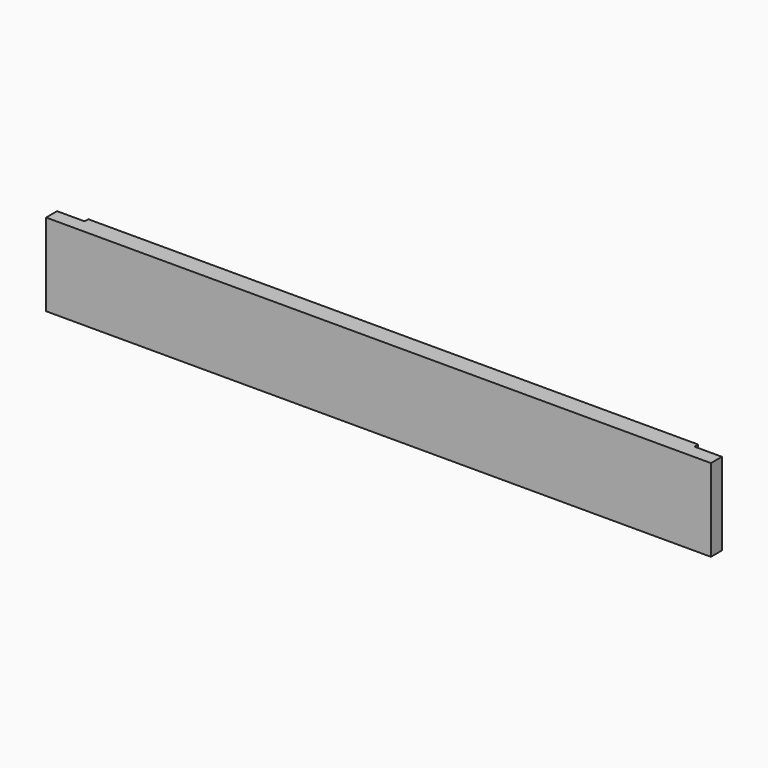
from build123d import *

# Parameters (mm, degrees)
F1_DEPTH      = 230.1875
F2_W          = 19.05
F2_H          = 9.525
F3_DEPTH      = 493
F3_DEPTH_BACK = 57.151


# Not quite as in the source:
# - an extrude ends at something that could not be found from the text; its depth is read off the source's solid


with BuildPart() as f1:
    # F0 (on Right) → F1 (new body, symmetric)
    with BuildSketch(Plane.YZ):
        Polygon((-19.05, 57.15), (-19.05, 0), (0, 0), (0, 38.1), (-6.35, 38.1), (-6.35, 57.15), align=None)
    extrude(amount=F1_DEPTH, both=True)

    # F2 (on Top) → F3 (cut, two sides)
    with BuildSketch(Plane.XY) as f3_sk:
        with Locations((220.6625, -4.7625)):
            Rectangle(F2_W, F2_H)
        with Locations((-220.6625, -4.7625)):
            Rectangle(F2_W, F2_H)
    extrude(amount=-F3_DEPTH, mode=Mode.SUBTRACT)
    extrude(f3_sk.sketch, amount=F3_DEPTH_BACK, mode=Mode.SUBTRACT)


solid = f1.part
